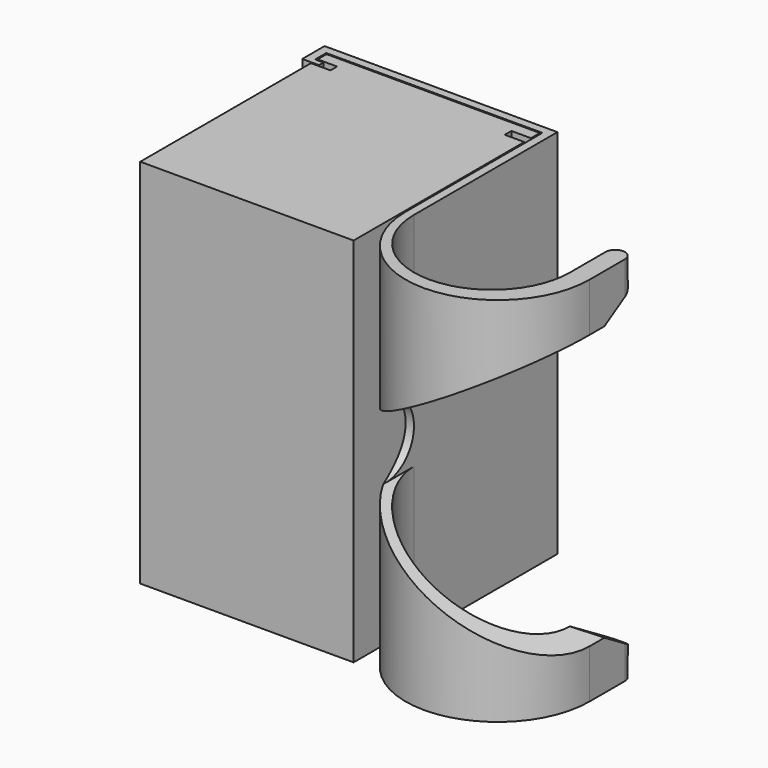
from build123d import *

# Parameters (mm, degrees)
F3_DEPTH = 133.35
F5_DEPTH = 97.3703234473
F7_DEPTH = 83.601
F9_DEPTH = 63


with BuildPart() as f3:
    # F1 (on Top) → F3 (new body)
    with BuildSketch(Plane.XY):
        Polygon((38.3, -2), (38.3, 2), (-38.3, 2), (-38.3, -2), (-31.3, -1.9999996343), (-31.3, -4.9999996343), (-38.3, -4.9999996343), (-38.3, -81.5999996343), (38.3, -81.5999996343), (38.3, -4.9999996343), (31.3, -4.9999996343), (31.3, -1.9999996343), align=None)
    extrude(amount=F3_DEPTH)


with BuildPart() as f3b:
    # F2 (on Top) → F3, piece 2 (new body)
    with BuildSketch(Plane.XY):
        with BuildLine():
            Line((-41.8, -4.4999996343), (-35.8, -4.4999996343))
            Line((-35.8, -4.4999996343), (-35.8, -2.5000000261))
            Line((-35.8, -2.5000000261), (-38.8, -2.5000000261))
            Line((-38.8, -2.5000000261), (-38.8, 2.5))
            Line((-38.8, 2.5), (38.8, 2.5))
            Line((38.8, 2.5), (38.8, -58.8693234473))
            ThreePointArc((38.8, -58.8693234473), (71.8, -91.8693234473), (104.8, -58.8693234473))
            Line((104.8, -58.8693234473), (104.8, -42.9086722434))
            ThreePointArc((104.8, -42.9086722434), (101.3, -39.4086722434), (97.8, -42.9086722434))
            Line((97.8, -42.9086722434), (97.8, -58.8693234473))
            ThreePointArc((97.8, -58.8693234473), (69.8, -86.8693234473), (41.8, -58.8693234473))
            Line((41.8, -58.8693234473), (41.8, 5.5))
            Line((41.8, 5.5), (-41.8, 5.5))
            Line((-41.8, 5.5), (-41.8, -4.4999996343))
        make_face()
    extrude(amount=F3_DEPTH)

    # F4 (on face) → F5 (cut, through all)
    with BuildSketch(Plane(origin=(0, 5.5, 0), x_dir=(-1, 0, 0), z_dir=(0, 1, 0))):
        Polygon((-41.8, 79.5144330411), (-104.8, 115.8875), (-104.8, 17.4625), (-41.8, 53.8355669589), align=None)
    extrude(amount=-F5_DEPTH, mode=Mode.SUBTRACT)

    # F6 (on face) → F7 (cut, through all)
    with BuildSketch(Plane.YZ.offset(41.8)):
        with BuildLine():
            Line((-72.6170505322, 79.5144330411), (-72.6170505322, 53.8355669589))
            ThreePointArc((-72.6170505322, 53.8355669589), (-58.8693234473, 66.675), (-72.6170505322, 79.5144330411))
        make_face()
    extrude(amount=-F7_DEPTH, mode=Mode.SUBTRACT)

    # F8 (on face) → F9 (cut, through all)
    with BuildSketch(Plane.YZ.offset(104.8)):
        Polygon((-39.4086722434, 113.8667740578), (-39.4086722434, 123.6083870289), (-58.8693234473, 111.8460481157), (-39.4086722434, 111.8460481157), align=None)
        Polygon((-58.8693234473, 21.5039518843), (-39.4086722434, 9.7416129711), (-39.4086722434, 19.4832259422), (-39.4086722434, 21.5039518843), align=None)
    extrude(amount=-F9_DEPTH, mode=Mode.SUBTRACT)


solid = Compound([f3.part, f3b.part])
